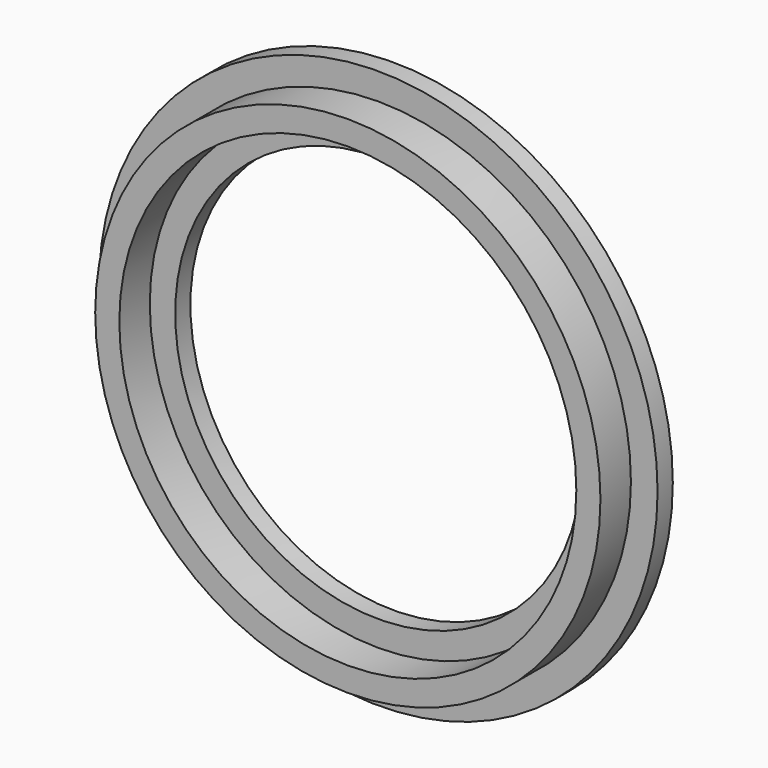
from build123d import *

# Parameters (mm, degrees)
F0_R     = 22
F0_R_2   = 16
F1_DEPTH = 1.5
F2_R     = 19.9
F2_R_2   = 18
F3_DEPTH = 3


# Not quite as in the source:
# - a feature names something its author has since deleted; it is built from what else it names


with BuildPart() as f1:
    # F0 (on Front) → F1 (new body)
    with BuildSketch(Plane.XZ):
        Circle(F0_R)
        Circle(F0_R_2, mode=Mode.SUBTRACT)
    extrude(amount=F1_DEPTH)

    # F2 (on face) → F3 (join)
    with BuildSketch(Plane.XZ.offset(1.5)):
        Circle(F2_R)
        Circle(F2_R_2, mode=Mode.SUBTRACT)
    extrude(amount=F3_DEPTH)


solid = f1.part
